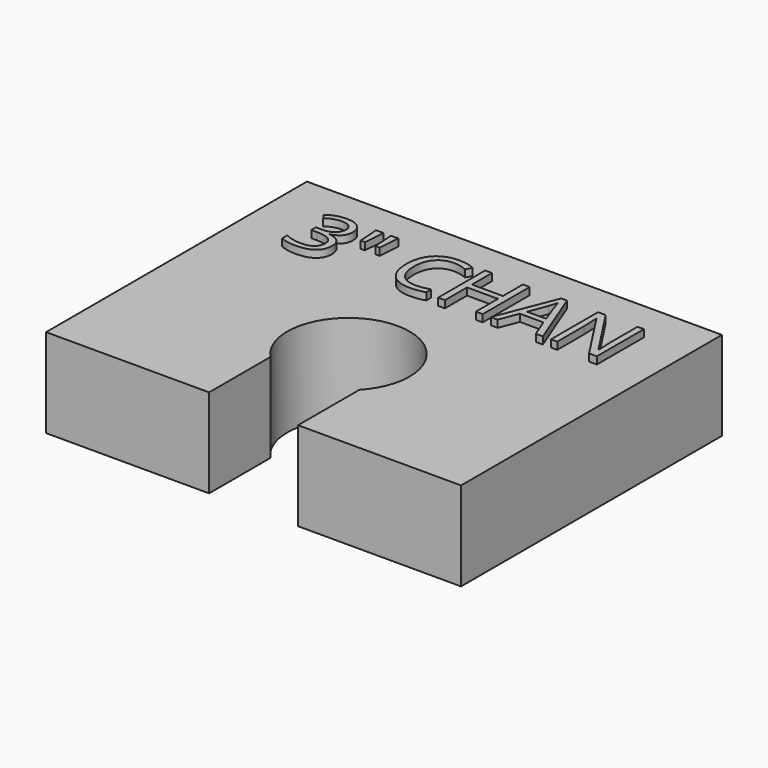
from build123d import *

# Parameters (mm, degrees)
F0_W         = 88.9
F0_H         = 69.85
F1_DEPTH     = 19.05
F3_DEPTH     = 25.4
F4_TEXT_SIZE = 17.6388888889
F5_DEPTH     = 1.5494


# Not quite as in the source:
# - Text() gives the source's letters only with a copy of the font that has no kerning and outlines rounded to 1/6400 em; it was checked with that copy


with BuildPart() as f1:
    # F0 (on Top) → F1 (new body)
    with BuildSketch(Plane.XY):
        with Locations((-8.6369048804, 14.2642892237)):
            Rectangle(F0_W, F0_H)
    extrude(amount=F1_DEPTH)

    # F2 (on face) → F3 (cut)
    with BuildSketch(Plane.XY.offset(19.05)):
        with BuildLine():
            Line((0.8880951196, -20.6607107763), (0.8880951196, -4.2497324008))
            ThreePointArc((0.8880951196, -4.2497324008), (-8.6369048804, 17.8361642237), (-18.1619048804, -4.2497324008))
            Line((-18.1619048804, -4.2497324008), (-18.1619048804, -20.6607107763))
            Line((-18.1619048804, -20.6607107763), (0.8880951196, -20.6607107763))
        make_face()
    extrude(amount=-F3_DEPTH, mode=Mode.SUBTRACT)

    # F4 (on face) → F5 (join)
    with BuildSketch(Plane.XY.offset(19.05)):
        with Locations((-42.4252338707, 27.7320992529)):
            Text('3" CHAN', F4_TEXT_SIZE, font='Open Sans', text_align=(TextAlign.LEFT, TextAlign.BOTTOM))
    extrude(amount=F5_DEPTH)


solid = f1.part
